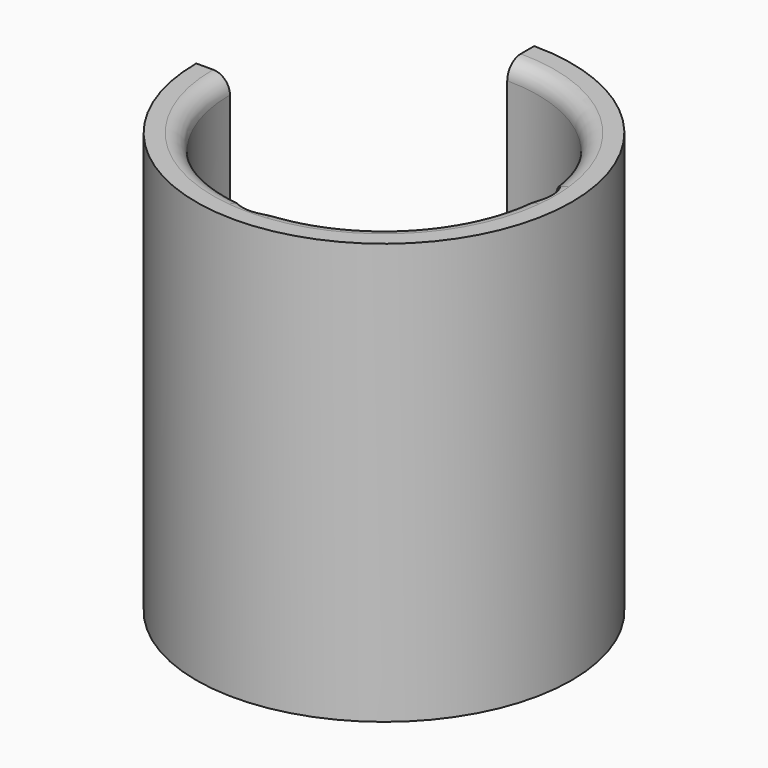
from build123d import *

# Parameters (mm, degrees)
F0_R         = 11.15
F1_DEPTH     = 25
F3_DEPTH     = 23
F4_T4_ANGLE  = 102.4463467312
F4_S5_R      = 1.65
F4_T6_DEPTH  = 9
F4_S7_R      = 1.65
F4_T8_DEPTH  = 9
F4_T12_ANGLE = 96.2242847007
F4_S13_R     = 1.65
F4_T14_DEPTH = 9
F4_T18_ANGLE = 96.2242847007
F4_S19_R     = 1.65
F4_T20_DEPTH = 9
F4_T22_ANGLE = 102.4463467312
F4_T24_ANGLE = 111.8839081247
F4_T26_ANGLE = 111.8839081247


# Not quite as in the source:
# - a fillet or chamfer that OpenCascade refuses, or shapes differently, is made with other operations: its cross-section is extruded or revolved along the edge and cut away or added


with BuildPart() as f1:
    # F0 (on Top) → F1 (new body)
    with BuildSketch(Plane.XY):
        Circle(F0_R)
    extrude(amount=F1_DEPTH)

    # F2 (on face) → F3 (cut)
    with BuildSketch(Plane.XY.offset(25)):
        with BuildLine():
            ThreePointArc((9.02621183, -1.5), (9.1190004453, -0.7525495849), (9.15, 0))
            ThreePointArc((9.15, 0), (9.1190004453, 0.7525495849), (9.02621183, 1.5))
            ThreePointArc((9.02621183, 1.5), (5.9159741379, 6.9802399672), (0, 9.15))
            ThreePointArc((0, 9.15), (-6.4700270479, 6.4700270479), (-9.15, 0))
            ThreePointArc((-9.15, 0), (-6.9802399672, -5.9159741379), (-1.5, -9.02621183))
            ThreePointArc((-1.5, -9.02621183), (0, -9.15), (1.5, -9.02621183))
            ThreePointArc((1.5, -9.02621183), (6.4700270479, -6.4700270479), (9.02621183, -1.5))
        make_face()
        with BuildLine():
            ThreePointArc((9.02621183, 1.5), (9.1190004453, 0.7525495849), (9.15, 0))
            ThreePointArc((9.15, 0), (9.1190004453, -0.7525495849), (9.02621183, -1.5))
            ThreePointArc((9.02621183, -1.5), (9.9888254758, 0), (9.02621183, 1.5))
        make_face()
        with BuildLine():
            ThreePointArc((-1.5, -9.02621183), (0, -9.9888254758), (1.5, -9.02621183))
            ThreePointArc((1.5, -9.02621183), (0, -9.15), (-1.5, -9.02621183))
        make_face()
        with BuildLine():
            ThreePointArc((-9.15, 0), (-6.4700270479, 6.4700270479), (0, 9.15))
            Line((0, 9.15), (0, 11.15))
            ThreePointArc((0, 11.15), (-7.8842406102, 7.8842406102), (-11.15, 0))
            Line((-11.15, 0), (-9.15, 0))
        make_face()
    extrude(amount=-F3_DEPTH, mode=Mode.SUBTRACT)

    # F4: fillet of radius 1 on 6 edges, made by hand


with BuildPart() as f4_tool2:
    # F4_s3 → F4_t4 (revolve)
    with BuildSketch(Plane(origin=(0, 0, 0), x_dir=(0, 0, 1), z_dir=(-0.9941072022, 0.1084014327, 0))):
        with BuildLine():
            ThreePointArc((2, -8.15), (2.2928932188, -8.8571067812), (3, -9.15))
            Line((3, -9.15), (2, -9.15))
            Line((2, -9.15), (2, -8.15))
        make_face()
    revolve(axis=Axis((0, 0, 2), (0, 0, 1)), revolution_arc=F4_T4_ANGLE)

    # F4_s5 → F4_t6 (cut, symmetric)
    with BuildSketch(Plane.XY.offset(2.9)):
        with Locations((8.3388254758, 0)):
            Circle(F4_S5_R)
    extrude(amount=F4_T6_DEPTH, both=True, mode=Mode.SUBTRACT)

    # F4_s7 → F4_t8 (cut, symmetric)
    with BuildSketch(Plane.XY.offset(2.9)):
        with Locations((0, -8.3388254758)):
            Circle(F4_S7_R)
    extrude(amount=F4_T8_DEPTH, both=True, mode=Mode.SUBTRACT)


with BuildPart() as f1_1:
    add(f1.part)

    # F4_t1: union F4_tool2
    add(f4_tool2.part)


with BuildPart() as f4_tool10:
    # F4_s11 → F4_t12 (revolve)
    with BuildSketch(Plane(origin=(0, 0, 0), x_dir=(0, 0, 1), z_dir=(-0.1084207149, -0.9941050994, 0))):
        with BuildLine():
            ThreePointArc((2, -8.15), (2.2928932188, -8.8571067812), (3, -9.15))
            Line((3, -9.15), (2, -9.15))
            Line((2, -9.15), (2, -8.15))
        make_face()
    revolve(axis=Axis((0, 0, 2), (0, 0, 1)), revolution_arc=F4_T12_ANGLE)

    # F4_s13 → F4_t14 (cut, symmetric)
    with BuildSketch(Plane.XY.offset(2.9)):
        with Locations((8.3388254758, 0)):
            Circle(F4_S13_R)
    extrude(amount=F4_T14_DEPTH, both=True, mode=Mode.SUBTRACT)


with BuildPart() as f1_2:
    add(f1_1.part)

    # F4_t9: union F4_tool10
    add(f4_tool10.part)


with BuildPart() as f4_tool16:
    # F4_s17 → F4_t18 (revolve)
    with BuildSketch(Plane.XZ):
        with BuildLine():
            ThreePointArc((-8.15, 2), (-8.8571067812, 2.2928932188), (-9.15, 3))
            Line((-9.15, 3), (-9.15, 2))
            Line((-9.15, 2), (-8.15, 2))
        make_face()
    revolve(axis=Axis((0, 0, 2), (0, 0, 1)), revolution_arc=F4_T18_ANGLE)

    # F4_s19 → F4_t20 (cut, symmetric)
    with BuildSketch(Plane.XY.offset(2.9)):
        with Locations((0, -8.3388254758)):
            Circle(F4_S19_R)
    extrude(amount=F4_T20_DEPTH, both=True, mode=Mode.SUBTRACT)


with BuildPart() as f1_3:
    add(f1_2.part)

    # F4_t15: union F4_tool16
    add(f4_tool16.part)

    # F4_s21 → F4_t22 (revolve, cut)
    with BuildSketch(Plane(origin=(0, 0, 0), x_dir=(0, 0, 1), z_dir=(-0.9941072022, 0.1084014327, 0))):
        with BuildLine():
            ThreePointArc((24, -9.15), (24.7071067812, -9.4428932188), (25, -10.15))
            Line((25, -10.15), (25, -9.15))
            Line((25, -9.15), (24, -9.15))
        make_face()
    revolve(axis=Axis((0, 0, 25), (0, 0, 1)), revolution_arc=F4_T22_ANGLE, mode=Mode.SUBTRACT)

    # F4_s23 → F4_t24 (revolve, cut)
    with BuildSketch(Plane(origin=(0, 0, 0), x_dir=(0, 0, 1), z_dir=(0.2699219659, 0.9628822006, 0))):
        with BuildLine():
            ThreePointArc((24, -9.15), (24.7071067812, -9.4428932188), (25, -10.15))
            Line((25, -10.15), (25, -9.15))
            Line((25, -9.15), (24, -9.15))
        make_face()
    revolve(axis=Axis((0, 0, 25), (0, 0, 1)), revolution_arc=F4_T24_ANGLE, mode=Mode.SUBTRACT)

    # F4_s25 → F4_t26 (revolve, cut)
    with BuildSketch(Plane(origin=(0, 0, 0), x_dir=(0, 0, 1), z_dir=(-0.1084207149, -0.9941050994, 0))):
        with BuildLine():
            ThreePointArc((24, -9.15), (24.7071067812, -9.4428932188), (25, -10.15))
            Line((25, -10.15), (25, -9.15))
            Line((25, -9.15), (24, -9.15))
        make_face()
    revolve(axis=Axis((0, 0, 25), (0, 0, 1)), revolution_arc=F4_T26_ANGLE, mode=Mode.SUBTRACT)


solid = f1_3.part
